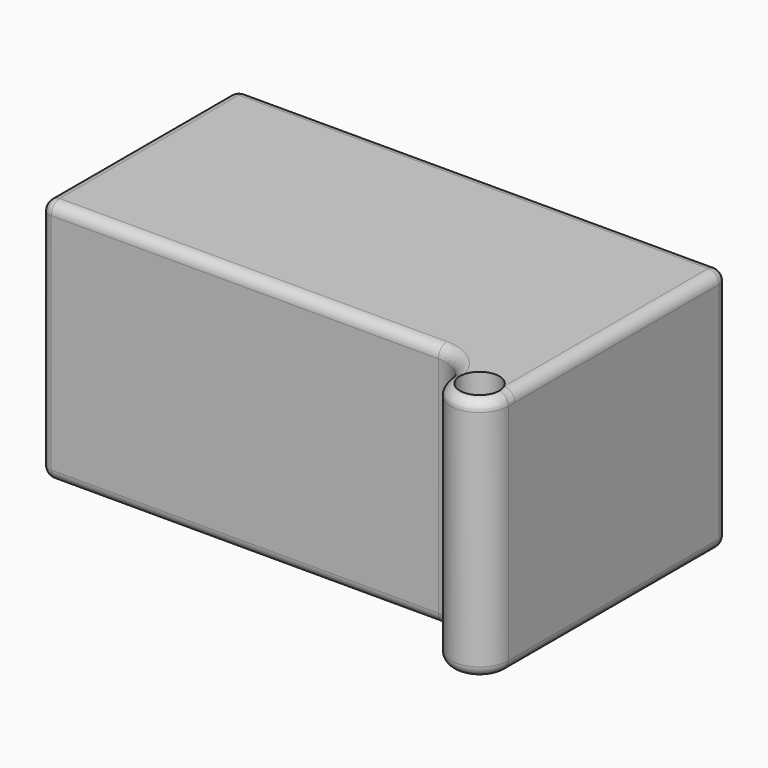
from build123d import *

# Parameters (mm, degrees)
F1_DEPTH             = 34.2
F2_W                 = 34.2
F2_H                 = 34.2
F3_DEPTH             = 34.2
F4_W                 = 28.2
F4_H                 = 28.2
F5_DEPTH             = 31.2
F8_D                 = 3.3
F8_DEPTH             = 25
F8_CSINK_D           = 6.72
F8_CSINK_ANGLE       = 90
F8_TIP               = 0.9914200214
F8_ON_F7_D           = 3.3
F8_ON_F7_DEPTH       = 25
F8_ON_F7_CSINK_D     = 6.72
F8_ON_F7_CSINK_ANGLE = 90
F8_ON_F7_TIP         = 0.9914200214
F10_D                = 5.5
F10_DEPTH            = 25
F10_TIP              = 1.6523667023
F11_R                = 5
F12_W                = 28.2
F12_H                = 28.2
F13_DEPTH            = 31.2
F14_R                = 1.49999


# Not quite as in the source:
# - a fillet or chamfer is up to 0.001 mm smaller than in the source, because OpenCascade refuses the exact size


with BuildPart() as f1:
    # F0 (on Top) → F1 (new body)
    with BuildSketch(Plane.XY):
        with BuildLine():
            Line((0, 0), (-8, 0))
            Line((-8, 0), (-8, -4))
            ThreePointArc((-8, -4), (-4, -8), (0, -4))
            Line((0, -4), (0, 0))
        make_face()
        Polygon((-34.2, 0), (-8, 0), (0, 0), (0, 34.2), (-34.2, 34.2), align=None)
    extrude(amount=F1_DEPTH)

    # F2 (on face) → F3 (join)
    with BuildSketch(Plane(origin=(-34.2, 0, 0), x_dir=(0, -1, 0), z_dir=(-1, 0, 0))):
        with Locations((-17.1, 17.1)):
            Rectangle(F2_W, F2_H)
    extrude(amount=F3_DEPTH)

    # F4 (on face) → F5 (cut)
    with BuildSketch(Plane(origin=(-68.4, 0, 0), x_dir=(0, -1, 0), z_dir=(-1, 0, 0))):
        with Locations((-17.1, 17.1)):
            Rectangle(F4_W, F4_H)
    extrude(amount=-F5_DEPTH, mode=Mode.SUBTRACT)

    # F8
    with Locations(Plane(origin=(0, 34.2, 0), x_dir=(-1, 0, 0), z_dir=(0, 1, 0))):
        with Locations((17.05, 17.1), (51.35, 17.1)):
            CounterSinkHole(F8_D / 2, F8_CSINK_D / 2, depth=F8_DEPTH, counter_sink_angle=F8_CSINK_ANGLE)
            with Locations((0, 0, -(F8_DEPTH + F8_TIP / 2))):  # 118° drill point
                Cone(0, F8_D / 2, F8_TIP, mode=Mode.SUBTRACT)

    # F8 on F7
    with Locations(Plane(origin=(-37.2, 0, 0), x_dir=(0, -1, 0), z_dir=(-1, 0, 0))):
        with Locations((-17.1, 17.1)):
            CounterSinkHole(F8_ON_F7_D / 2, F8_ON_F7_CSINK_D / 2, depth=F8_ON_F7_DEPTH, counter_sink_angle=F8_ON_F7_CSINK_ANGLE)
            with Locations((0, 0, -(F8_ON_F7_DEPTH + F8_ON_F7_TIP / 2))):  # 118° drill point
                Cone(0, F8_ON_F7_D / 2, F8_ON_F7_TIP, mode=Mode.SUBTRACT)

    # F10
    with Locations(Plane.XY.offset(34.2)):
        with Locations((-4, -4)):
            Hole(F10_D / 2, depth=F10_DEPTH)
            with Locations((0, 0, -(F10_DEPTH + F10_TIP / 2))):  # 118° drill point
                Cone(0, F10_D / 2, F10_TIP, mode=Mode.SUBTRACT)

    # F11
    f11_edges = [f1.edges().sort_by_distance(p)[0] for p in [
        (-8, 0, 17.1),
    ]]
    fillet(f11_edges, radius=F11_R)

    # F12 (on face) → F13 (cut)
    with BuildSketch(Plane(origin=(0, 0, 0), x_dir=(1, 0, 0), z_dir=(0, 0, -1))):
        with Locations((-17.1, -17.1)):
            Rectangle(F12_W, F12_H)
    extrude(amount=-F13_DEPTH, mode=Mode.SUBTRACT)

    # F14 (radius 1.5 in the source; OpenCascade refuses exactly that, so slightly less here)
    f14_edges = [f1.edges().sort_by_distance(p)[0] for p in [
        (-31.2, 17.1, 0),
        (-17.1, 3, 0),
        (-3, 17.1, 0),
        (-17.1, 31.2, 0),
        (-34.2, 34.2, 0),
        (-40.672136, 0, 0),
        (0, 15.1, 0),
        (-68.4, 17.1, 0),
        (-68.4, 0, 17.1),
        (-68.4, 17.1, 34.2),
        (-68.4, 34.2, 17.1),
        (-68.4, 17.1, 31.2),
        (-68.4, 3, 17.1),
        (-68.4, 17.1, 3),
        (-68.4, 31.2, 17.1),
        (-40.672136, 0, 34.2),
        (-34.2, 34.2, 34.2),
        (0, 15.1, 34.2),
        (0, 34.2, 17.1),
    ]]
    fillet(f14_edges, radius=F14_R)


solid = f1.part
